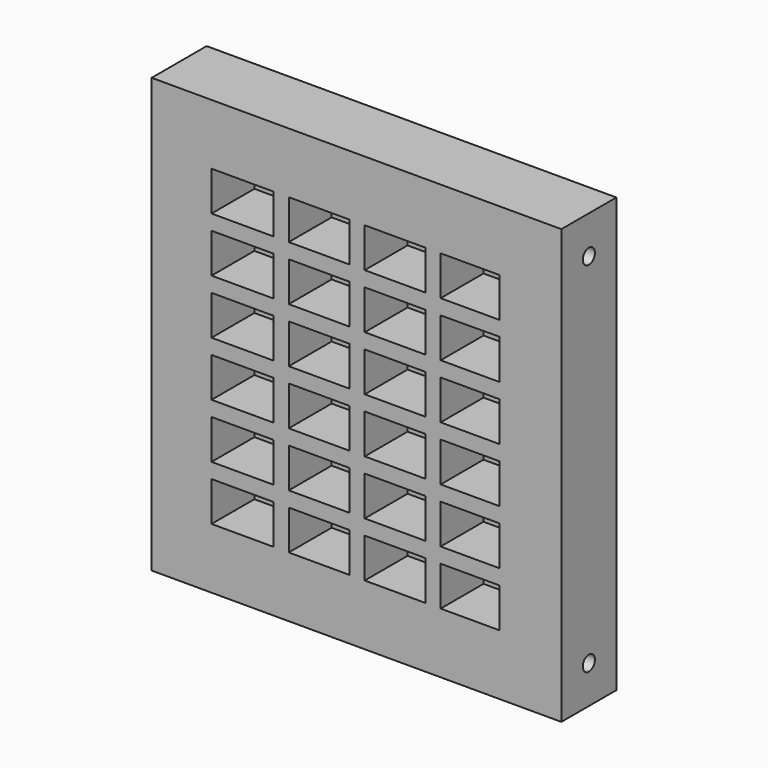
from build123d import *

# Parameters (mm, degrees)
F0_W     = 171.958
F0_H     = 182.0672
F0_W_2   = 25.527
F0_H_2   = 16.5862
F1_DEPTH = 28.829
F0_W_3   = 24.7371567947
F2_DEPTH = 6.35
F3_R     = 3.175
F4_DEPTH = 203.2


# Not quite as in the source:
# - a length typed as a fraction of an inch, garbled in the dataset ("3 / 203.2 mm" for 3/8 in), is restored


with BuildPart() as f1:
    # F0 (on Front) → F1 (new body)
    with BuildSketch(Plane.XZ):
        with Locations((85.979, -91.0336)):
            Rectangle(F0_W, F0_H)
        Polygon((25.1346008565, -41.4550490677), (25.1346008565, -25.4), (51.1923991435, -25.4), (57.5423991435, -25.4), (83.0693991435, -25.4), (85.5840783974, -25.4), (89.4193991435, -25.4), (114.9463991435, -25.4), (121.2963991435, -25.4), (146.0335559382, -25.4), (146.0335559382, -41.9862), (146.0335559382, -48.1976613704), (146.0335559382, -64.9224), (146.0335559382, -71.2724), (146.0335559382, -87.8586), (146.0335559382, -94.2086), (146.0335559382, -110.7948), (146.0335559382, -117.1448), (146.0335559382, -133.731), (146.0335559382, -140.081), (146.0335559382, -156.6672), (121.2963991435, -156.6672), (114.9463991435, -156.6672), (89.4193991435, -156.6672), (83.0693991435, -156.6672), (57.5423991435, -156.6672), (51.1923991435, -156.6672), (25.1346008565, -156.6672), (25.1346008565, -140.081), (25.1346008565, -133.731), (25.1346008565, -117.1448), (25.1346008565, -110.7948), (25.1346008565, -94.2086), (25.1346008565, -87.8586), (25.1346008565, -71.2724), (25.1346008565, -64.9224), (25.1346008565, -48.3362), (25.1346008565, -41.9862), align=None, mode=Mode.SUBTRACT)
        Polygon((57.5423991435, -25.4), (51.1923991435, -25.4), (51.1923991435, -41.9862), (25.1346008565, -41.9862), (25.1346008565, -48.3362), (38.1635, -48.3362), (51.1923991435, -48.3362), (51.1923991435, -64.9224), (38.1635, -64.9224), (25.1346008565, -64.9224), (25.1346008565, -71.2724), (38.1635, -71.2724), (51.1923991435, -71.2724), (51.1923991435, -87.8586), (38.1635, -87.8586), (25.1346008565, -87.8586), (25.1346008565, -94.2086), (38.1635, -94.2086), (51.1923991435, -94.2086), (51.1923991435, -110.7948), (25.1346008565, -110.7948), (25.1346008565, -117.1448), (38.1635, -117.1448), (51.1923991435, -117.1448), (51.1923991435, -133.731), (38.1635, -133.731), (25.1346008565, -133.731), (25.1346008565, -140.081), (38.1635, -140.081), (51.1923991435, -140.081), (51.1923991435, -156.6672), (57.5423991435, -156.6672), (57.5423991435, -140.081), (83.0693991435, -140.081), (83.0693991435, -156.6672), (89.4193991435, -156.6672), (89.4193991435, -140.081), (114.9463991435, -140.081), (114.9463991435, -156.6672), (121.2963991435, -156.6672), (121.2963991435, -140.081), (146.0335559382, -140.081), (146.0335559382, -133.731), (121.2963991435, -133.731), (121.2963991435, -117.1448), (146.0335559382, -117.1448), (146.0335559382, -110.7948), (121.2963991435, -110.7948), (121.2963991435, -94.2086), (146.0335559382, -94.2086), (146.0335559382, -87.8586), (121.2963991435, -87.8586), (121.2963991435, -71.2724), (146.0335559382, -71.2724), (146.0335559382, -64.9224), (121.2963991435, -64.9224), (121.2963991435, -48.3362), (146.0335559382, -48.1976613704), (146.0335559382, -41.9862), (121.2963991435, -41.9862), (121.2963991435, -25.4), (114.9463991435, -25.4), (114.9463991435, -41.9862), (89.4193991435, -41.9862), (89.4193991435, -25.4), (85.5840783974, -25.4), (83.0693991435, -25.4), (83.0693991435, -41.9862), (57.5423991435, -41.9862), align=None)
        with Locations((70.3058991435, -125.4379)):
            Rectangle(F0_W_2, F0_H_2, mode=Mode.SUBTRACT)
        with Locations((70.3058991435, -102.5017)):
            Rectangle(F0_W_2, F0_H_2, mode=Mode.SUBTRACT)
        with Locations((102.1828991435, -125.4379)):
            Rectangle(F0_W_2, F0_H_2, mode=Mode.SUBTRACT)
        with Locations((102.1828991435, -102.5017)):
            Rectangle(F0_W_2, F0_H_2, mode=Mode.SUBTRACT)
        with Locations((70.3058991435, -79.5655)):
            Rectangle(F0_W_2, F0_H_2, mode=Mode.SUBTRACT)
        with Locations((70.3058991435, -56.6293)):
            Rectangle(F0_W_2, F0_H_2, mode=Mode.SUBTRACT)
        with Locations((102.1828991435, -79.5655)):
            Rectangle(F0_W_2, F0_H_2, mode=Mode.SUBTRACT)
        with Locations((102.1828991435, -56.6293)):
            Rectangle(F0_W_2, F0_H_2, mode=Mode.SUBTRACT)
    extrude(amount=F1_DEPTH)

    # F0 (on Front) → F2 (join)
    with BuildSketch(Plane.XZ):
        Polygon((51.1923991435, -25.4), (25.1346008565, -25.4), (25.1346008565, -41.4550490677), (25.1346008565, -41.9862), (51.1923991435, -41.9862), align=None)
        with Locations((70.3058991435, -33.6931)):
            Rectangle(F0_W_2, F0_H_2)
        with Locations((102.1828991435, -33.6931)):
            Rectangle(F0_W_2, F0_H_2)
        with Locations((133.6649775409, -33.6931)):
            Rectangle(F0_W_3, F0_H_2)
        Polygon((146.0335559382, -64.9224), (146.0335559382, -48.1976613704), (121.2963991435, -48.3362), (121.2963991435, -64.9224), align=None)
        with Locations((102.1828991435, -56.6293)):
            Rectangle(F0_W_2, F0_H_2)
        with Locations((70.3058991435, -56.6293)):
            Rectangle(F0_W_2, F0_H_2)
        Polygon((38.1635, -48.3362), (25.1346008565, -48.3362), (25.1346008565, -64.9224), (38.1635, -64.9224), (51.1923991435, -64.9224), (51.1923991435, -48.3362), align=None)
        Polygon((38.1635, -71.2724), (25.1346008565, -71.2724), (25.1346008565, -87.8586), (38.1635, -87.8586), (51.1923991435, -87.8586), (51.1923991435, -71.2724), align=None)
        with Locations((70.3058991435, -79.5655)):
            Rectangle(F0_W_2, F0_H_2)
        with Locations((102.1828991435, -79.5655)):
            Rectangle(F0_W_2, F0_H_2)
        with Locations((133.6649775409, -79.5655)):
            Rectangle(F0_W_3, F0_H_2)
        with Locations((133.6649775409, -102.5017)):
            Rectangle(F0_W_3, F0_H_2)
        with Locations((102.1828991435, -102.5017)):
            Rectangle(F0_W_2, F0_H_2)
        with Locations((70.3058991435, -102.5017)):
            Rectangle(F0_W_2, F0_H_2)
        Polygon((38.1635, -94.2086), (25.1346008565, -94.2086), (25.1346008565, -110.7948), (51.1923991435, -110.7948), (51.1923991435, -94.2086), align=None)
        Polygon((38.1635, -117.1448), (25.1346008565, -117.1448), (25.1346008565, -133.731), (38.1635, -133.731), (51.1923991435, -133.731), (51.1923991435, -117.1448), align=None)
        with Locations((133.6649775409, -125.4379)):
            Rectangle(F0_W_3, F0_H_2)
        with Locations((133.6649775409, -148.3741)):
            Rectangle(F0_W_3, F0_H_2)
        with Locations((102.1828991435, -148.3741)):
            Rectangle(F0_W_2, F0_H_2)
        with Locations((70.3058991435, -148.3741)):
            Rectangle(F0_W_2, F0_H_2)
        Polygon((38.1635, -140.081), (25.1346008565, -140.081), (25.1346008565, -156.6672), (51.1923991435, -156.6672), (51.1923991435, -140.081), align=None)
        with Locations((102.1828991435, -125.4379)):
            Rectangle(F0_W_2, F0_H_2)
        with Locations((70.3058991435, -125.4379)):
            Rectangle(F0_W_2, F0_H_2)
    extrude(amount=F2_DEPTH)

    # F3 (on face) → F4 (cut)
    with BuildSketch(Plane(origin=(0, 0, 0), x_dir=(0, -1, 0), z_dir=(-1, 0, 0))):
        with Locations((14.4145, -15.875)):
            Circle(F3_R)
        with Locations((14.4145, -166.1922)):
            Circle(F3_R)
    extrude(amount=-F4_DEPTH, mode=Mode.SUBTRACT)


solid = f1.part
